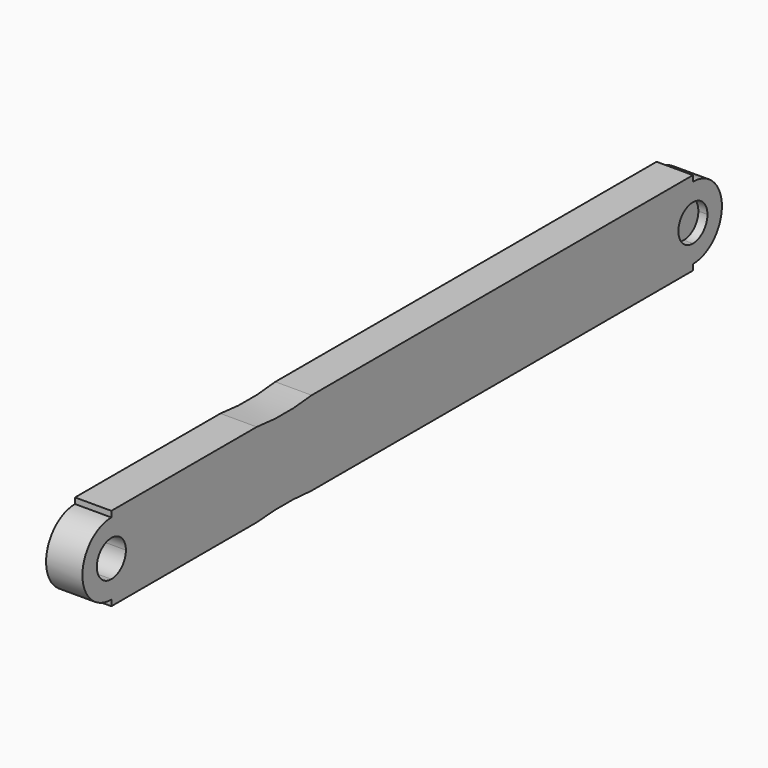
from build123d import *

# Parameters (mm, degrees)
F1_DEPTH = 25.4
F2_R     = 12.7
F3_DEPTH = 19.05


with BuildPart() as f1:
    # F0 (on Right) → F1 (new body)
    with BuildSketch(Plane.YZ):
        with BuildLine():
            Line((90.1355675816, 48.1937031183), (-36.8644324184, 48.1937031183))
            Line((-36.8644324184, 48.1937031183), (-36.8644324184, 44.1192870285))
            ThreePointArc((-36.8644324184, 44.1192870285), (-18.9902183288, 36.7155451359), (-11.5864764361, 18.8413310463))
            ThreePointArc((-11.5864764361, 18.8413310463), (-18.9902183288, 0.9671169568), (-36.8644324184, -6.4366249359))
            Line((-36.8644324184, -6.4366249359), (-36.8644324184, -10.5110410257))
            Line((-36.8644324184, -10.5110410257), (90.1355675816, -10.5110410257))
            ThreePointArc((90.1355675816, -10.5110410257), (114.1056831658, -9.2312943557), (138.0757987499, -10.5110410257))
            Line((138.0757987499, -10.5110410257), (471.1355675816, -10.5110410257))
            Line((471.1355675816, -10.5110410257), (471.1355675816, -6.490723888))
            ThreePointArc((471.1355675816, -6.490723888), (445.8035126474, 18.8413310463), (471.1355675816, 44.1733859806))
            Line((471.1355675816, 44.1733859806), (471.1355675816, 48.1937031183))
            Line((471.1355675816, 48.1937031183), (138.0757987499, 48.1937031183))
            ThreePointArc((138.0757987499, 48.1937031183), (114.1056831658, 46.5243458888), (90.1355675816, 48.1937031183))
        make_face()
        with BuildLine():
            ThreePointArc((-11.5864764361, 18.8413310463), (-18.9902183288, 36.7155451359), (-36.8644324184, 44.1192870285))
            Line((-36.8644324184, 44.1192870285), (-36.8644324184, 31.5413310463))
            ThreePointArc((-36.8644324184, 31.5413310463), (-27.8841762973, 27.8215871674), (-24.1644324184, 18.8413310463))
            ThreePointArc((-24.1644324184, 18.8413310463), (-27.8841762973, 9.8610749252), (-36.8644324184, 6.1413310463))
            Line((-36.8644324184, 6.1413310463), (-36.8644324184, -6.4366249359))
            ThreePointArc((-36.8644324184, -6.4366249359), (-18.9902183288, 0.9671169568), (-11.5864764361, 18.8413310463))
        make_face()
        with BuildLine():
            Line((-36.8644324184, 31.5413310463), (-36.8644324184, 44.1192870285))
            ThreePointArc((-36.8644324184, 44.1192870285), (-62.1423884006, 18.8413310463), (-36.8644324184, -6.4366249359))
            Line((-36.8644324184, -6.4366249359), (-36.8644324184, 6.1413310463))
            ThreePointArc((-36.8644324184, 6.1413310463), (-49.5644324184, 18.8413310463), (-36.8644324184, 31.5413310463))
        make_face()
        with BuildLine():
            ThreePointArc((496.4676225159, 18.8413310463), (489.0480354071, 36.7537988717), (471.1355675816, 44.1733859806))
            Line((471.1355675816, 44.1733859806), (471.1355675816, 31.5413310463))
            ThreePointArc((471.1355675816, 31.5413310463), (480.1158237027, 27.8215871674), (483.8355675816, 18.8413310463))
            ThreePointArc((483.8355675816, 18.8413310463), (480.1158237027, 9.8610749252), (471.1355675816, 6.1413310463))
            Line((471.1355675816, 6.1413310463), (471.1355675816, -6.490723888))
            ThreePointArc((471.1355675816, -6.490723888), (489.0480354071, 0.9288632209), (496.4676225159, 18.8413310463))
        make_face()
        with BuildLine():
            Line((471.1355675816, 31.5413310463), (471.1355675816, 44.1733859806))
            ThreePointArc((471.1355675816, 44.1733859806), (445.8035126474, 18.8413310463), (471.1355675816, -6.490723888))
            Line((471.1355675816, -6.490723888), (471.1355675816, 6.1413310463))
            ThreePointArc((471.1355675816, 6.1413310463), (458.4355675816, 18.8413310463), (471.1355675816, 31.5413310463))
        make_face()
    extrude(amount=F1_DEPTH)


with BuildPart() as f3:
    # F2 (on face) → F3 (new body, symmetric)
    with BuildSketch(Plane(origin=(0, 0, 0), x_dir=(0, -1, 0), z_dir=(-1, 0, 0))):
        with Locations((-471.1355675816, 18.8413310463)):
            Circle(F2_R)
    extrude(amount=F3_DEPTH, both=True)


solid = Compound([f1.part, f3.part])
